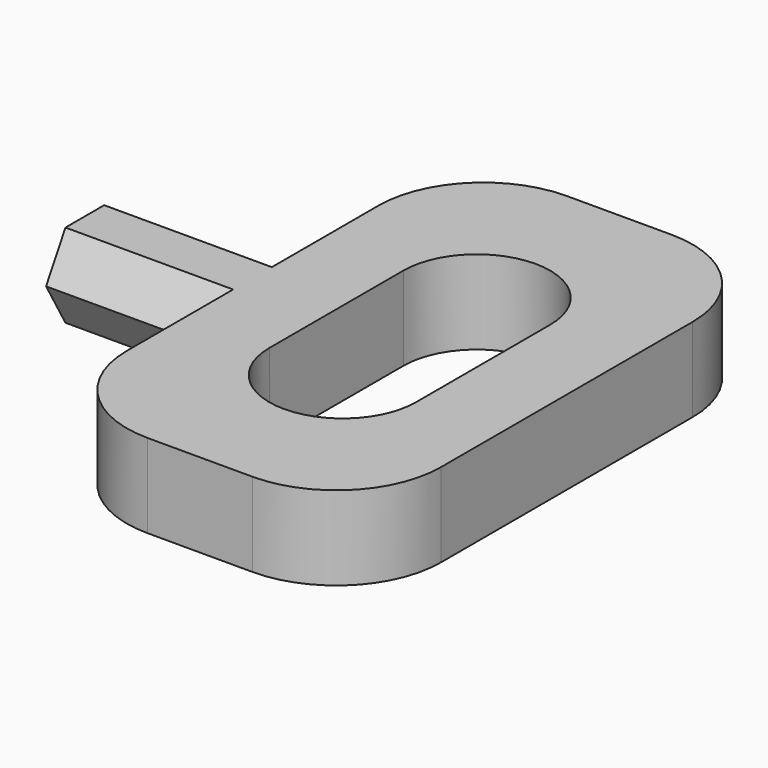
from build123d import *

# Parameters (mm, degrees)
F0_W     = 15
F0_H     = 25
F1_DEPTH = 4
F3_DEPTH = 8
F5_DEPTH = 4
F6_R     = 5


# Not quite as in the source:
# - a feature names something its author has since deleted; it is built from what else it names


with BuildPart() as f1:
    # F0 (on Top) → F1 (new body)
    with BuildSketch(Plane.XY):
        with Locations((38.2812308715, -12.5)):
            Rectangle(F0_W, F0_H)
    extrude(amount=F1_DEPTH)

    # F2 (on face) → F3 (join)
    with BuildSketch(Plane(origin=(30.7812308715, 0, 0), x_dir=(0, -1, 0), z_dir=(-1, 0, 0))):
        Polygon((13.6547005384, 0), (14.8094010768, 2), (13.6547005384, 4), (11.3452994616, 4), (10.1905989232, 2), (11.3452994616, 0), align=None)
    extrude(amount=F3_DEPTH)

    # F4 (on face) → F5 (cut, through all)
    with BuildSketch(Plane.XY.offset(4)):
        with BuildLine():
            Line((34.7812308715, -16.5), (41.7812308715, -16.5))
            ThreePointArc((41.7812308715, -16.5), (38.2812308715, -13), (34.7812308715, -16.5))
        make_face()
        with BuildLine():
            ThreePointArc((34.7812308715, -16.5), (38.2812308715, -20), (41.7812308715, -16.5))
            Line((41.7812308715, -16.5), (34.7812308715, -16.5))
        make_face()
        with BuildLine():
            ThreePointArc((34.7812308715, -16.5), (38.2812308715, -13), (41.7812308715, -16.5))
            Line((41.7812308715, -16.5), (41.7812308715, -8.5))
            ThreePointArc((41.7812308715, -8.5), (38.2812308715, -12), (34.7812308715, -8.5))
            Line((34.7812308715, -8.5), (34.7812308715, -16.5))
        make_face()
        with BuildLine():
            Line((34.7812308715, -8.5), (41.7812308715, -8.5))
            ThreePointArc((41.7812308715, -8.5), (38.2812308715, -5), (34.7812308715, -8.5))
        make_face()
        with BuildLine():
            ThreePointArc((34.7812308715, -8.5), (38.2812308715, -12), (41.7812308715, -8.5))
            Line((41.7812308715, -8.5), (34.7812308715, -8.5))
        make_face()
    extrude(amount=-F5_DEPTH, mode=Mode.SUBTRACT)

    # F6
    f6_edges = [f1.edges().sort_by_distance(p)[0] for p in [
        (45.781231, 0, 2),
        (30.781231, 0, 2),
        (45.781231, -25, 2),
        (30.781231, -25, 2),
    ]]
    fillet(f6_edges, radius=F6_R)


solid = f1.part
